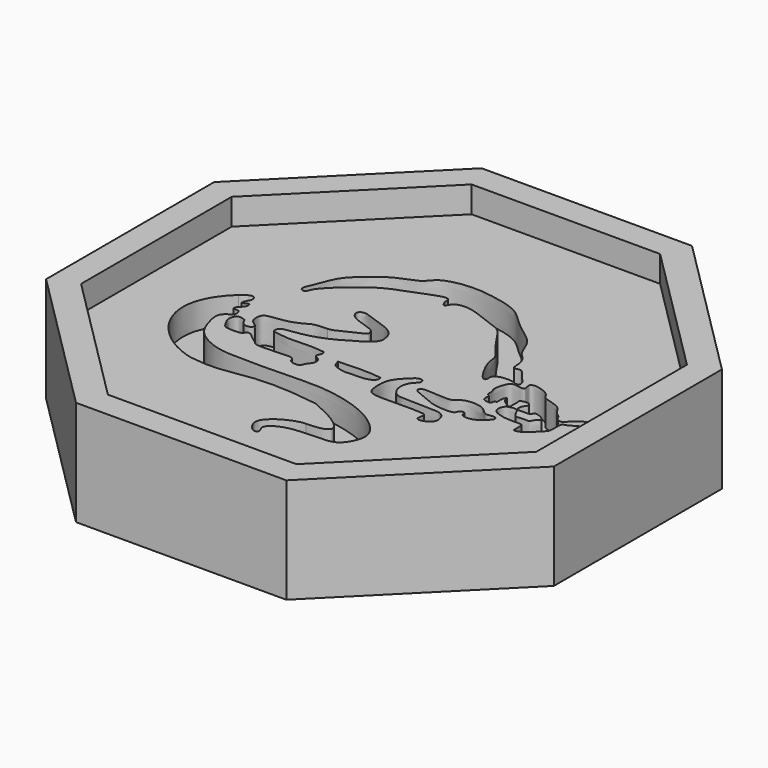
from build123d import *

# Parameters (mm, degrees)
F1_DEPTH = 25.4
F3_DEPTH = 6.35
F5_DEPTH = 6.35


with BuildPart() as f1:
    # F0 (on Top) → F1 (new body)
    with BuildSketch(Plane.XY):
        Polygon((-61.3372846899, 25.3607087968), (-61.3047391097, -25.4392807779), (-25.3607087968, -61.3372846899), (25.4392807779, -61.3047391097), (61.3372846899, -25.3607087968), (61.3047391097, 25.4392807779), (25.3607087968, 61.3372846899), (-25.4392807779, 61.3047391097), align=None)
    extrude(amount=F1_DEPTH)

    # F2 (on face) → F3 (cut)
    with BuildSketch(Plane.XY.offset(25.4)):
        Polygon((-54.9856008905, 22.734521413), (-54.9564255154, -22.8049569991), (-22.734521413, -54.9856008905), (22.8049569991, -54.9564255154), (54.9856008905, -22.734521413), (54.9564255154, 22.8049569991), (22.734521413, 54.9856008905), (-22.8049569991, 54.9564255154), align=None)
    extrude(amount=-F3_DEPTH, mode=Mode.SUBTRACT)

    # F4 (on face) → F5 (cut)
    with BuildSketch(Plane.XY.offset(19.05)):
        with BuildLine():
            add(Edge.make_bspline(
                [(-28.8479506651, 11.9264236432), (-28.9179859332, 11.5456937254), (-28.8673623906, 10.7682750421), (-27.4197242632, 10.6381749719), (-27.4003946424, 12.8773237618), (-18.9408746635, 20.2486089262), (-14.7009780752, 22.0244412287), (-7.7860965591, 24.6523686611), (-5.9661656974, 25.3501676819), (-4.227714812, 25.2847315843), (-4.5866641258, 23.9099401432), (-3.4408224811, 22.0018377815), (-2.8352584057, 24.3517363715), (-0.0471699757, 24.8766592038), (3.0958860634, 24.1945838088), (6.8189167073, 22.4704643041), (10.6126887593, 21.5531811585), (12.4061703924, 18.3282335766), (15.4437878377, 14.2789173273), (17.529548232, 11.9396916102), (17.0597769186, 9.5356755609), (20.8111740209, 2.9344716579), (21.6977234704, 4.4081689953), (21.2936460797, 5.3617689972), (22.8553837572, 6.7258614285), (26.3797801501, 6.5611101787), (26.9191136989, 5.9214975088), (28.0161061695, 6.2585177778), (27.4750730398, 7.7744631474), (25.7531299791, 9.173292223), (24.6260329973, 11.2202741494), (23.3797167425, 10.9504587482), (22.3826798753, 10.6769366778), (22.4549428957, 12.785868539), (21.7519133744, 15.0743503276), (19.9085918359, 16.2490508976), (19.0324100731, 19.0938819385), (17.6065570763, 21.5621370818), (14.6997503022, 23.5850584693), (11.3584355478, 26.2055625657), (8.3244129072, 29.6376827228), (2.0803916106, 31.2065139176), (-4.3929613808, 32.0542469157), (-11.0467189543, 30.6671274004), (-12.6474095024, 27.8594554869), (-14.7754535992, 27.0470388939), (-19.2383329577, 25.2487171537), (-22.7746942524, 22.1591478213), (-26.3137124068, 19.2101847022), (-28.0011199027, 13.7631645395), (-28.7515709696, 12.4503687143), (-28.8479506651, 11.9264236432)],
                knots=[0, 0, 0, 0, 0.0122343745, 0.0237629786, 0.0395590072, 0.0791570167, 0.1079173221, 0.1398885137, 0.1573948355, 0.1707573723, 0.1841199011, 0.1986691076, 0.2135068964, 0.233079904, 0.2549908202, 0.2797555979, 0.3029865784, 0.3258480018, 0.353527931, 0.3738066602, 0.3935196714, 0.4243262457, 0.4345137039, 0.4460070003, 0.4621724692, 0.4845114223, 0.4950839842, 0.5056565461, 0.5191305347, 0.5379315066, 0.5555962819, 0.5683025959, 0.5784387279, 0.5943563218, 0.6132617764, 0.6306155434, 0.6511166305, 0.6714979121, 0.6941072895, 0.7191235184, 0.7447340102, 0.7748961886, 0.8067796725, 0.8374359478, 0.8578108619, 0.8755629172, 0.9019457048, 0.9284334419, 0.9546115111, 0.9831635501, 1, 1, 1, 1], degree=3))
        make_face()
        with BuildLine():
            add(Edge.make_bspline(
                [(-36.5214720368, 1.7604259774), (-36.1759309845, 2.1845827823), (-35.283486355, 2.7215409174), (-33.7187972779, 3.383769561), (-33.1520827364, 1.622751516), (-33.7127305986, 1.223570816), (-34.5239139109, -1.0545138585), (-33.1877441821, 0.1219542662), (-32.3505863369, 0.1799137966), (-32.5009597592, -0.9852953215), (-32.7482517867, -1.4287164779), (-33.6490550006, -2.0849601398), (-34.0892516023, -3.1947332944), (-33.1958379518, -3.2470390342), (-32.0773556682, -3.1456660592), (-32.0397891659, -5.1733361641), (-32.631550474, -5.3087613371), (-34.8633115759, -6.5679057738), (-34.4535162704, -8.8280664884), (-34.0225279013, -10.1745148408)],
                knots=[0, 0, 0, 0, 0.0699013277, 0.1332735037, 0.1956924403, 0.244440349, 0.3126257492, 0.3684302835, 0.4119515491, 0.4643679084, 0.5045732117, 0.5625605006, 0.6143647044, 0.6584445206, 0.7109661686, 0.7793015705, 0.8192350544, 0.8977226931, 1, 1, 1, 1], degree=3))
            add(Edge.make_bspline(
                [(-36.5214720368, 1.7604259774), (-48.0737090111, -8.8955170941), (-38.1096556464, -21.4356371421), (-27.5533042529, -23.8257573205)],
                knots=[0, 0, 0, 0, 27.1123737278, 27.1123737278, 27.1123737278, 27.1123737278], degree=3))
            add(Edge.make_bspline(
                [(-27.5533042529, -23.8257573205), (-16.6981845775, -25.5187564749), (-16.3994181583, -20.9376962143), (2.5223480391, -23.8257573205)],
                knots=[0, 0, 0, 0, 30.075652292, 30.075652292, 30.075652292, 30.075652292], degree=3))
            add(Edge.make_bspline(
                [(2.5223480391, -23.8257573205), (7.4021721577, -25.7179347086), (17.560173603, -31.1952886391), (6.2071129998, -31.3944650102)],
                knots=[0, 0, 0, 0, 8.4180062311, 8.4180062311, 8.4180062311, 8.4180062311], degree=3))
            add(Edge.make_bspline(
                [(6.2071129998, -31.3944650102), (3.4186421747, -31.3944650102), (-2.7558290547, -34.6808769959), (-1.5607704788, -37.5689381021)],
                knots=[0, 0, 0, 0, 9.9229094373, 9.9229094373, 9.9229094373, 9.9229094373], degree=3))
            add(Edge.make_bspline(
                [(-1.5607704788, -37.5689381021), (-1.3840096952, -37.9789415378), (-1.0188193779, -38.8259935465), (0.3639765233, -40.0199914901), (1.3518388209, -39.5234465955), (1.0576225936, -38.5616651208), (0.4051173917, -37.4960892715), (1.9598386515, -35.766094566), (5.692176611, -34.4567037027), (11.2317007067, -34.4467416414), (15.1034678317, -34.2640933246), (17.0332932501, -32.5583152042), (18.5660409335, -29.4095862962), (18.0642212884, -26.3031736124), (14.6964743346, -22.9522692813), (9.7474436656, -20.1149750379), (0.4608095272, -17.6417945885), (-9.9766728904, -18.2626864921), (-20.7936813701, -18.2648164232), (-26.7124805624, -17.935807816), (-32.4829333545, -14.763964409), (-33.6369509803, -11.6620747964), (-34.0225279013, -10.1745148408)],
                knots=[0, 0, 0, 0, 0.0301868303, 0.0630418862, 0.0852253352, 0.1088010454, 0.1353712886, 0.1704095305, 0.2211697658, 0.2821034354, 0.3312484706, 0.3705648182, 0.4169778221, 0.460436172, 0.5141519773, 0.5750790116, 0.6529642455, 0.7370251643, 0.8203543594, 0.8826056284, 0.9451671389, 1, 1, 1, 1], degree=3))
        make_face()
        with BuildLine():
            add(Edge.make_bspline(
                [(-29.2774449715, -5.5082101594), (-29.1586827354, -5.8283459657), (-28.9149084194, -6.4854646738), (-28.0309767429, -7.3197139013), (-26.4639174989, -7.1732619636), (-25.9715328573, -6.1049105448), (-27.5004261599, -5.31006053), (-28.2046516815, -4.2484707598), (-28.1479365448, -1.6158820027), (-25.5441487812, -1.3426742614), (-23.002152661, -1.0488857886), (-19.7204462298, 0.0875610324), (-18.1681379502, 1.3532480266), (-16.00917566, 1.4071255127), (-14.7876005301, 1.4376102495)],
                knots=[0, 0, 0, 0, 0.0627189205, 0.1287384142, 0.2021522623, 0.2571870772, 0.3320065784, 0.4033660678, 0.4934172067, 0.5847471757, 0.6876026747, 0.8009922334, 0.8873982471, 1, 1, 1, 1], degree=3))
            add(Edge.make_bspline(
                [(-29.2774449715, -5.5082101594), (-29.984591732, -5.2433040835), (-31.3369692763, -4.7363808543), (-32.045024307, -6.6874333745), (-31.9131583734, -7.567936275), (-31.0345764716, -9.1488425895), (-30.2449642716, -10.312431066), (-27.4080620237, -10.2031958311), (-26.2777941322, -10.12439348), (-25.6507971187, -8.9637861059), (-24.5757276432, -9.3174635805), (-23.830332584, -10.2265245363), (-22.0992906389, -11.2238369181), (-21.3547395187, -12.6138120403), (-13.098962532, -11.4482474338), (-12.1878881252, -12.399984623), (-12.1237042484, -13.5000844033), (-9.5749342627, -13.8240020305), (-9.2806996062, -12.7289912083), (-8.672290109, -11.6924875985), (-7.9618635542, -10.9658515676), (-8.0655892049, -9.5538142709), (-9.0801510147, -8.8750883196), (-9.8859124341, -8.633465727), (-9.0590817269, -7.1269357157), (-9.3691159985, -6.3235504445), (-10.1511398793, -6.3826315335), (-12.3596025644, -5.950144549), (-17.806111158, -6.4769352096), (-21.0428878765, -5.8452606317), (-22.273402119, -5.6679407488), (-22.2343552944, -4.6992193258), (-21.5590105618, -3.7860290399), (-18.4637105597, -3.5604039805), (-13.8836049347, -2.6158020833), (-10.1356480152, -0.7914105283), (-8.4067510122, 0.3741349806)],
                knots=[0, 0, 0, 0, 0.0311588295, 0.0595894337, 0.0813888382, 0.110978859, 0.1370607789, 0.1738393298, 0.1977770982, 0.2209525721, 0.2420901833, 0.2670367617, 0.297723875, 0.3248382914, 0.3880820831, 0.4112861042, 0.4322094033, 0.4646893202, 0.4866585415, 0.5112538414, 0.5336343594, 0.5586948032, 0.5831598748, 0.6004935758, 0.6278615674, 0.6466330239, 0.6641814134, 0.6973711851, 0.75109388, 0.7925322498, 0.8145268912, 0.8338048817, 0.8559531908, 0.8940487825, 0.9435897797, 1, 1, 1, 1], degree=3))
            add(Edge.make_bspline(
                [(-14.7876005301, 1.4376102495), (-14.4807171011, 1.4616653313), (-13.5164156561, 1.5372521762), (-8.497515223, 4.1069787382), (-7.3025612359, 4.6761863856), (-7.8850158443, 6.1407837346), (-9.2969723545, 6.689153271), (-14.1317632328, 8.0509743278), (-14.9121323908, 10.2523905763), (-13.3756784976, 11.1581202608), (-11.0548312017, 10.1396951332), (-7.4933611118, 9.1845261649), (-4.4659816214, 7.5362776323), (-3.868270781, 5.4542119714), (-3.6697111589, 3.4187433443), (-6.5435526663, 1.3494148445), (-7.8307477636, 0.6756403846), (-8.4067510122, 0.3741349806)],
                knots=[0, 0, 0, 0, 0.0485833605, 0.152660588, 0.1991738518, 0.2456002288, 0.300352892, 0.3973739027, 0.4548652575, 0.5039132273, 0.5716561042, 0.6575194872, 0.7365748872, 0.7981053151, 0.856813306, 0.9359257962, 1, 1, 1, 1], degree=3))
        make_face()
        with BuildLine():
            add(Edge.make_bspline(
                [(-4.9021054672, -7.7999281916), (-1.3582783665, -7.6134112883), (2.2228521614, -7.4455455165), (5.5615099466, -7.9304903033)],
                knots=[0, 0, 0, 0, 10.4644299411, 10.4644299411, 10.4644299411, 10.4644299411], degree=3))
            add(Edge.make_bspline(
                [(5.5615099466, -7.9304903033), (5.600594571, -8.3621324059), (5.692715788, -9.3794991168), (3.2532032727, -10.293129017), (0.6335931075, -10.0910972035), (-1.3831663343, -10.4234639013), (-3.1100104717, -9.9207344817), (-4.4768619316, -9.3860359177), (-4.7569551781, -8.3413214774), (-4.9021054672, -7.7999281916)],
                knots=[0, 0, 0, 0, 0.1174764518, 0.2768882615, 0.4527906216, 0.6035820489, 0.7444592647, 0.8675733454, 1, 1, 1, 1], degree=3))
        make_face()
        with BuildLine():
            add(Edge.make_bspline(
                [(10.1910595169, -4.4877455789), (10.5641270258, -4.1338321521), (10.9935919471, -3.7407846339), (12.2827266571, -3.4365110023), (12.7964753034, -4.7096636278), (11.8980073348, -5.3839568745), (10.6935331339, -6.8709130648), (10.5584071047, -9.5224307418), (12.297222136, -11.9575815513), (15.5442086877, -11.6322748887), (19.9357184569, -12.0632023954), (23.2016136863, -11.8219009832), (24.7359084997, -13.2972697905), (24.9248596496, -15.7612151612), (23.0158463791, -16.7787475022), (21.1163106929, -16.9923935791), (21.3873039833, -15.595095896), (21.5903296092, -14.447536817), (20.3750647226, -14.2528926326), (17.8378196233, -14.1375537423), (13.1164927874, -14.2954853597), (8.2339408614, -14.2638363578), (7.1390408357, -12.7418922462), (6.9618218028, -9.9718707397), (7.3724540322, -7.2055890338), (9.527809567, -5.116942861), (10.1910595169, -4.4877455789)],
                knots=[0, 0, 0, 0, 0.0307419325, 0.0598084741, 0.087996854, 0.1161852292, 0.1548411573, 0.2000902907, 0.2454659894, 0.2949606549, 0.355829307, 0.4061740564, 0.4447789217, 0.4858362356, 0.526390295, 0.5606508523, 0.5902030626, 0.6187095522, 0.6457818758, 0.6907098433, 0.7546914024, 0.8159016031, 0.8510765715, 0.8970907091, 0.9453461244, 1, 1, 1, 1], degree=3))
        make_face()
        with BuildLine():
            add(Edge.make_bspline(
                [(21.7924312076, -6.5767384353), (21.1407566683, -6.874768428), (19.0436034971, -6.5967735724), (14.6381512715, -6.411577217), (14.047076083, -6.8786801697), (13.9909416837, -7.8491638056), (15.8427431243, -8.3772913431), (19.7668028002, -10.4112191937), (22.881289078, -10.605476417), (25.5073270234, -10.5470616434), (25.4813882147, -9.2780551238), (27.1410957854, -8.8705444938), (26.8200427725, -10.2839210098), (28.1083664873, -10.6355561713), (30.0811716029, -10.4441375782), (31.8212289824, -9.1008851441), (33.1455587322, -7.6139342742), (32.4850389745, -6.8186398115), (30.9719138765, -7.1300127428), (30.0261581178, -7.2011819738), (28.7981703836, -5.8967639465), (27.7897300778, -5.2475700581), (25.6210655456, -4.8729908733), (23.0417792298, -5.2620572073), (22.3015391065, -6.3439083733), (21.7924312076, -6.5767384353)],
                knots=[0, 0, 0, 0, 0.0559707886, 0.1254060995, 0.1509310353, 0.1781862901, 0.2213322631, 0.2916959769, 0.3528625261, 0.4016255289, 0.4340750043, 0.4690074865, 0.5009351602, 0.5352856372, 0.5817832911, 0.6322686896, 0.6760959499, 0.7031818998, 0.7432959848, 0.7754430997, 0.8180451018, 0.8547842843, 0.9035472862, 0.9562739238, 1, 1, 1, 1], degree=3))
        make_face()
        with BuildLine():
            add(Edge.make_bspline(
                [(31.4037546834, -2.3448223933), (31.1833858274, -2.5212887141), (30.6314407614, -3.3396028636), (30.7964813187, -4.9177304987), (32.042029417, -5.6386939737), (34.0203705202, -6.1207175523), (34.4746822443, -6.0850666999), (36.2707363985, -6.3016671378), (38.3926148823, -6.0102769274), (38.431172371, -7.030532121), (38.4801082694, -8.1792380468), (38.4284010088, -9.0590797515), (39.2146312692, -8.986972757), (40.7972751326, -8.4402812671), (42.072710327, -6.8547154847), (43.746233173, -5.4205032477), (44.1538738142, -4.4395884783), (43.7796599389, -1.2295504172), (45.2695497192, -1.312649548), (47.2790533085, 0.3077418402), (49.0282873901, 0.4529081351), (48.4150664796, 2.2713688252), (47.5269890482, 2.5142720128), (45.7861985948, 1.4871707732), (44.3422296818, 0.1795956922), (43.7119682713, -0.6366463951), (42.9250386751, -0.7263008912), (42.0163970086, -0.2973833489), (41.6624229696, 0.805123988), (40.7693686705, 1.189303505), (39.932860361, 2.3680401104), (39.2619094666, 3.5616950251), (37.6442298298, 4.1711487556), (36.0417556311, 4.6491722137), (34.8340159121, 4.974359385), (34.1020529871, 6.6902045564), (31.7273438389, 7.5046805076), (30.3974517292, 7.814093202), (29.1915708137, 7.4071736061), (29.4681827882, 6.3364308118), (29.6334553736, 5.3727843142), (28.3364284968, 5.4148391225), (27.2354866677, 5.8049898704), (26.0834356678, 5.4686973381), (25.485022311, 4.1932895727), (24.8414712455, 1.8711500186), (25.6081844836, 0.7367773943), (25.3320504932, -0.8031895699), (26.3245613434, -0.8434219851), (26.0874538964, -1.6777878455), (26.1070793919, -2.508978899), (26.7091363959, -2.9408732398), (28.5066595008, -3.242404637), (28.1088219594, -1.9069410971), (29.0377894908, -2.1430301701), (28.6284813762, -0.8474819989), (29.3335256242, 0.9929147718), (29.4151408381, -0.3442956442), (30.0428442603, -0.9976235856), (30.741450235, -1.455042409), (31.6225256557, -2.1435534309), (32.0845024188, -1.7086697021), (31.7927500949, -1.0677225921), (32.1104126552, 0.1774399053), (31.6155279835, 1.1370379816), (33.3300092285, 1.5116572627), (34.1413413085, 1.326380082), (34.5377767837, 0.4711567114), (33.7407349885, -0.1630249749), (33.4812177361, -1.1810775207), (33.7648796023, -2.2527102317), (35.3771629163, -1.8824753934), (37.1717208927, -2.143953007), (36.9875512487, -0.9708075488), (38.6757278858, -1.2060332928), (39.571224002, -1.92765475), (40.0458910394, -2.3087148942), (39.3419454839, -3.0469597142), (38.8168885521, -3.5272526798), (38.6427672995, -4.4469522898), (37.1345333716, -4.1205371149), (35.5180243594, -4.5486146841), (34.8536842466, -3.9057299011), (34.2473424525, -2.9357184822), (34.0073840314, -2.0613233979), (32.8348177805, -1.8353168253), (31.8499773684, -2.1681434865), (31.5447358999, -2.2319278717), (31.4037546834, -2.3448223933)],
                knots=[0, 0, 0, 0, 0.0118046448, 0.0248251904, 0.0378377929, 0.0530862119, 0.0605889285, 0.0753356327, 0.0904579246, 0.0997555642, 0.1119957644, 0.1211138192, 0.1293298486, 0.1432836456, 0.1592283292, 0.175004344, 0.186623549, 0.2046873172, 0.2160429723, 0.2336975894, 0.2465082722, 0.2593998852, 0.2689487958, 0.2842071035, 0.2998309466, 0.3105024605, 0.3196205157, 0.3301561421, 0.3414274201, 0.3518849131, 0.3648398682, 0.3774995329, 0.3916168435, 0.4058897991, 0.4175401599, 0.4317646437, 0.4487873764, 0.4618458599, 0.4725972336, 0.4833739001, 0.4928577543, 0.5038279872, 0.5160085011, 0.5270523264, 0.5398746739, 0.5564471074, 0.5691973528, 0.5814831704, 0.590076833, 0.599152991, 0.6088436516, 0.6182442276, 0.6310798554, 0.6408504083, 0.6482341129, 0.6600131108, 0.6727498057, 0.6820013154, 0.6926338971, 0.7029824346, 0.713888377, 0.7208130943, 0.7294884264, 0.7418861144, 0.7515651989, 0.7645777974, 0.7746187635, 0.7837918012, 0.7941483593, 0.8053436467, 0.8152104725, 0.8287571824, 0.8423376047, 0.8511235395, 0.8638193244, 0.8760518778, 0.8831883521, 0.8932808498, 0.9029249568, 0.9119917252, 0.9246875101, 0.9386528973, 0.9484830312, 0.9601510896, 0.9700972312, 0.9813730431, 0.9924479656, 1, 1, 1, 1], degree=3))
        make_face()
    extrude(amount=-F5_DEPTH, mode=Mode.SUBTRACT)


solid = f1.part
